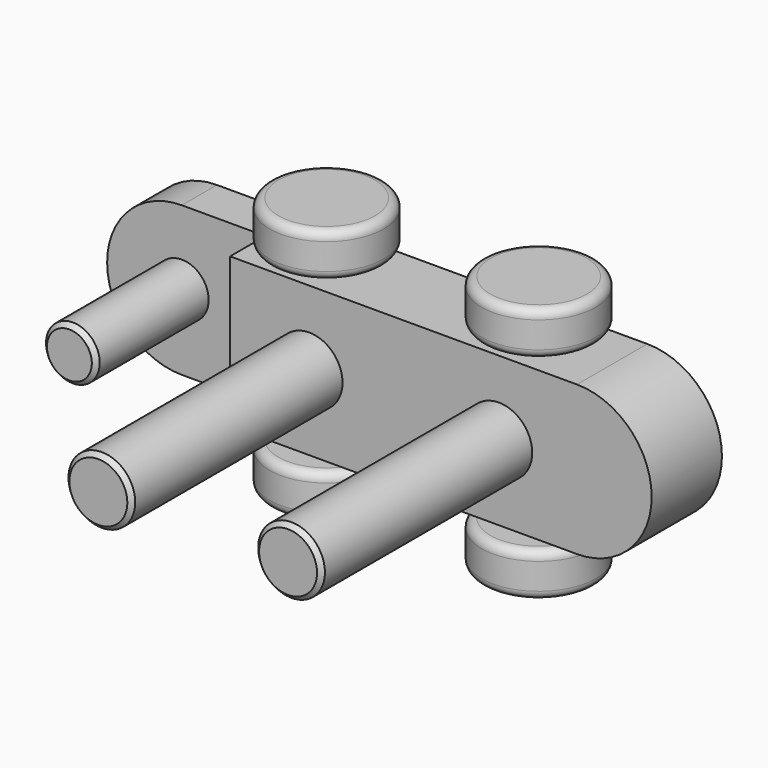
from build123d import *

# Parameters (mm, degrees)
F0_R      = 9.652
F1_DEPTH  = 25.4
F2_DEPTH  = 12.7
F3_DEPTH  = 101.6
F5_R      = 7.7669536028
F6_DEPTH  = 40.64
F4_R      = 8.3905783295
F7_DEPTH  = 43.181
F8_R      = 7.3745783295
F9_DEPTH  = 24.384
F10_R     = 16.51
F10_R_2   = 7.3745783295
F11_DEPTH = 12.7
F12_R     = 2.54
F12_2_R   = 2.54
F14_SIZE  = 1.27


# Not quite as in the source:
# - a feature names something its author has since deleted; it is built from what else it names


with BuildPart() as f1:
    # F0 (on Front) → F1 (new body)
    with BuildSketch(Plane.XZ):
        with BuildLine():
            Line((124.46, 21.59), (24.13, 21.59))
            Line((24.13, 21.59), (24.13, -21.59))
            Line((24.13, -21.59), (124.46, -21.59))
            ThreePointArc((124.46, -21.59), (146.05, 0), (124.46, 21.59))
        make_face()
        with Locations((46.99, 0)):
            Circle(F0_R, mode=Mode.SUBTRACT)
        with Locations((101.854, 0)):
            Circle(F0_R, mode=Mode.SUBTRACT)
    extrude(amount=F1_DEPTH)

    # F0 (on Front) → F2 (join)
    with BuildSketch(Plane.XZ):
        with BuildLine():
            Line((24.13, 21.59), (0, 21.59))
            ThreePointArc((0, 21.59), (-21.59, 0), (0, -21.59))
            Line((0, -21.59), (24.13, -21.59))
            Line((24.13, -21.59), (24.13, 21.59))
        make_face()
    extrude(amount=F2_DEPTH)

    # F0 (on Front) → F3 (join)
    with BuildSketch(Plane.XZ):
        with Locations((46.99, 0)):
            Circle(F0_R)
        with Locations((101.854, 0)):
            Circle(F0_R)
    extrude(amount=F3_DEPTH)

    # F5 (on face) → F6 (join)
    with BuildSketch(Plane.XZ.offset(12.7)):
        Circle(F5_R)
    extrude(amount=F6_DEPTH)

    # F4 (on face) → F7 (cut, through all)
    with BuildSketch(Plane(origin=(0, 0, -21.59), x_dir=(1, 0, 0), z_dir=(0, 0, -1))):
        with Locations((103.21611166, 12.7)):
            Circle(F4_R)
        with Locations((41.91, 12.7)):
            Circle(F4_R)
    extrude(amount=-F7_DEPTH, mode=Mode.SUBTRACT)

    # F14
    f14_edges = [f1.edges().sort_by_distance(p)[0] for p in [
        (92.202, -101.6, 0),
        (37.338, -101.6, 0),
        (-7.766954, -53.34, 0),
    ]]
    chamfer(f14_edges, length=F14_SIZE)


with BuildPart() as f9:
    # F8 (on Top) → F9 (new body, symmetric)
    with BuildSketch(Plane.XY):
        with Locations((41.91, -12.7)):
            Circle(F8_R)
    extrude(amount=F9_DEPTH, both=True)



with BuildPart() as f9b:
    # F8 (on Top) → F9, piece 2 (new body, symmetric)
    with BuildSketch(Plane.XY):
        with Locations((103.21611166, -12.7)):
            Circle(F8_R)
    extrude(amount=F9_DEPTH, both=True)


with BuildPart() as f11:
    # F10 (on face) → F11 (new body)
    with BuildSketch(Plane(origin=(0, 0, -24.384), x_dir=(1, 0, 0), z_dir=(0, 0, -1))):
        with Locations((41.91, 12.7)):
            Circle(F10_R)
        with Locations((41.91, 12.7)):
            Circle(F10_R_2, mode=Mode.SUBTRACT)
        with Locations((41.91, 12.7)):
            Circle(F10_R_2)
    extrude(amount=F11_DEPTH)

    # F12
    f12_edges = [f11.edges().sort_by_distance(p)[0] for p in [
        (25.4, -12.7, -37.084),
        (25.4, -12.7, -24.384),
    ]]
    fillet(f12_edges, radius=F12_R)


with BuildPart() as f11b:
    # F10 (on face) → F11, piece 2 (new body)
    with BuildSketch(Plane(origin=(0, 0, -24.384), x_dir=(1, 0, 0), z_dir=(0, 0, -1))):
        with Locations((103.21611166, 12.7)):
            Circle(F10_R)
    extrude(amount=F11_DEPTH)

    # F12#2
    f12_2_edges = [f11b.edges().sort_by_distance(p)[0] for p in [
        (86.706112, -12.7, -37.084),
        (86.706112, -12.7, -24.384),
    ]]
    fillet(f12_2_edges, radius=F12_2_R)


with BuildPart() as f9_1:
    add(f9.part)

    add(f9b.part)  # F13 merges F9b

    add(f11.part)  # F13 merges F11

    add(f11b.part)  # F13 merges F11b
    # F13: F9, F11, F11b, F9b across plane
    add(f9.part.mirror(Plane.XY))
    add(f11.part.mirror(Plane.XY))
    add(f11b.part.mirror(Plane.XY))
    add(f9b.part.mirror(Plane.XY))


solid = Compound([f1.part, f9_1.part])
